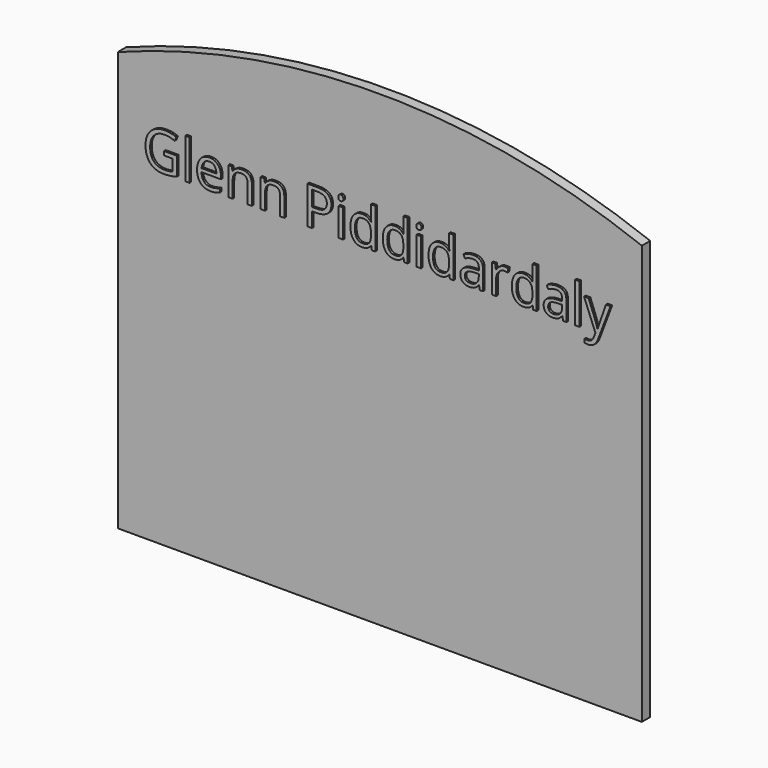
from build123d import *

# Parameters (mm, degrees)
F0_W         = 50
F0_H         = 40
F1_DEPTH     = 1
F2_TEXT_SIZE = 5.0392819023
F3_DEPTH     = 0.2


# Not quite as in the source:
# - Text() gives the source's letters only with a copy of the font that has no kerning and outlines rounded to 1/6400 em; it was checked with that copy


with BuildPart() as f1:
    # F0 (on Front) → F1 (new body)
    with BuildSketch(Plane.XZ):
        Rectangle(F0_W, F0_H)
        with BuildLine():
            Line((-25, 20), (25, 20))
            ThreePointArc((25, 20), (0, 24.6165158469), (-25, 20))
        make_face()
    extrude(amount=F1_DEPTH)

    # F2 (on face) → F3 (join)
    with BuildSketch(Plane.XZ.offset(1)):
        with Locations((-22.5, 11.3717170303)):
            Text('Glenn Piddidardaly', F2_TEXT_SIZE, font='Open Sans', text_align=(TextAlign.LEFT, TextAlign.BOTTOM))
    extrude(amount=F3_DEPTH)


solid = f1.part
